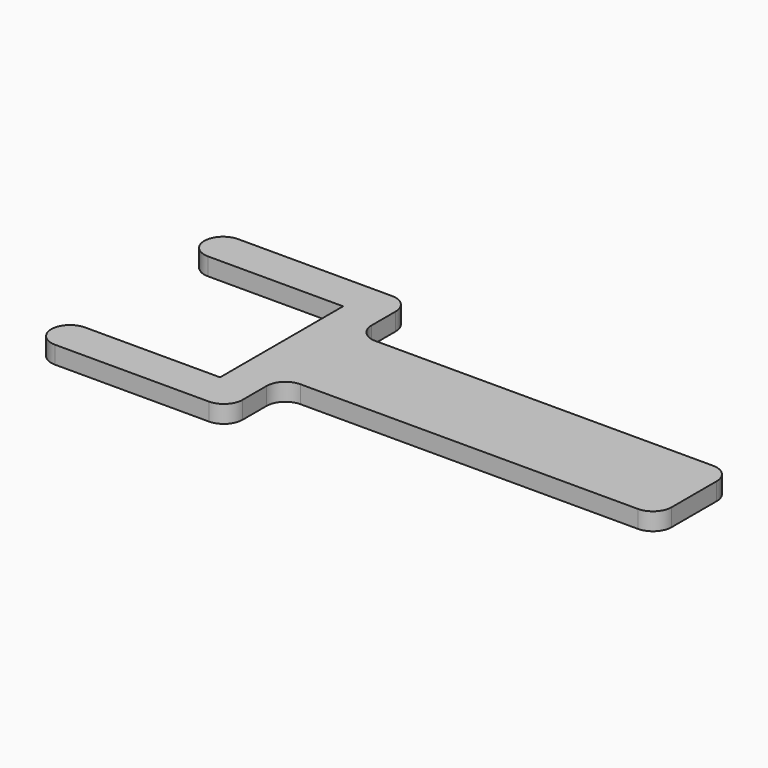
from build123d import *

# Parameters (mm, degrees)
F1_DEPTH = 4.7625
F2_R     = 5.07999


# Not quite as in the source:
# - a fillet or chamfer is up to 0.001 mm smaller than in the source, because OpenCascade refuses the exact size
# - a length typed as a fraction of an inch, garbled in the dataset ("3 / 203.2 mm" for 3/8 in), is restored


with BuildPart() as f1:
    # F0 (on Top) → F1 (new body)
    with BuildSketch(Plane.XY):
        Polygon((41.656, 0), (0, 0), (0, -10.16), (51.816, -10.16), (51.816, 8.128), (153.416, 8.128), (153.416, 33.528), (51.816, 33.528), (51.816, 51.816), (0, 51.816), (0, 41.656), (41.656, 41.656), align=None)
    extrude(amount=F1_DEPTH)

    # F2 (radius 5.08 in the source; OpenCascade refuses exactly that, so slightly less here)
    f2_edges = [f1.edges().sort_by_distance(p)[0] for p in [
        (0, 41.656, 2.38125),
        (0, 51.816, 2.38125),
        (0, 0, 2.38125),
        (0, -10.16, 2.38125),
        (51.816, -10.16, 2.38125),
        (51.816, 8.128, 2.38125),
        (51.816, 33.528, 2.38125),
        (51.816, 51.816, 2.38125),
        (153.416, 33.528, 2.38125),
        (153.416, 8.128, 2.38125),
    ]]
    fillet(f2_edges, radius=F2_R)


solid = f1.part
